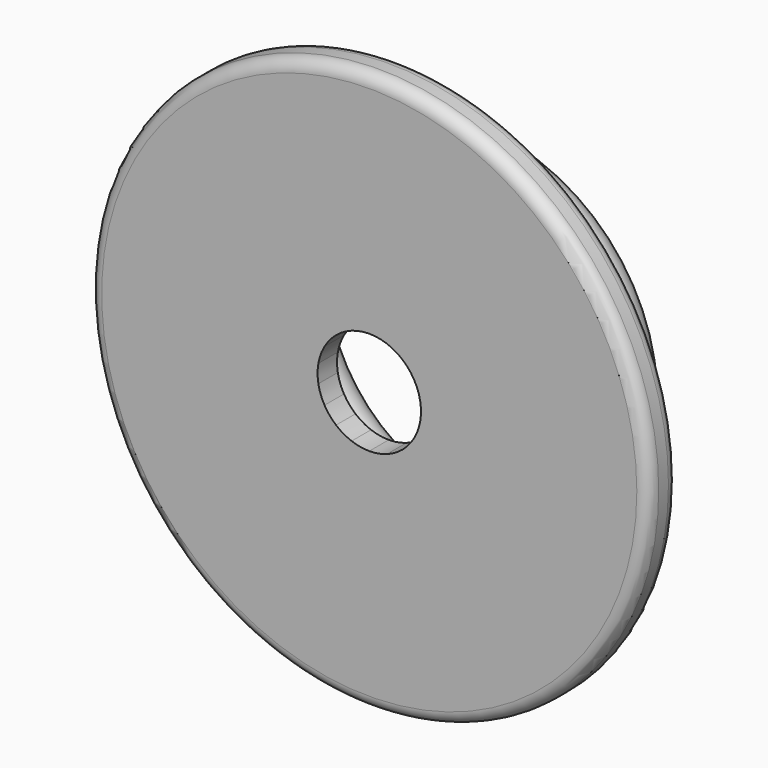
from build123d import *

# Parameters (mm, degrees)
F1_DEPTH = 10
F2_DEPTH = 2
F0_R     = 23
F3_DEPTH = 3
F4_DEPTH = 3.5
F5_R     = 1.6436802894
F7_R     = 1


with BuildPart() as f1:
    # F0 (on Front) → F1 (new body)
    with BuildSketch(Plane.XZ):
        with BuildLine():
            ThreePointArc((14.7721162952, -2.604722665), (14.9429204714, -1.3073361412), (15, 0))
            ThreePointArc((15, 0), (14.9429204714, 1.3073361412), (14.7721162952, 2.604722665))
            Line((14.7721162952, 2.604722665), (13.2949046657, 2.3442503985))
            ThreePointArc((13.2949046657, 2.3442503985), (13.4486284242, 1.1766025271), (13.5, 0))
            ThreePointArc((13.5, 0), (13.4486284242, -1.1766025271), (13.2949046657, -2.3442503985))
            Line((13.2949046657, -2.3442503985), (14.7721162952, -2.604722665))
        make_face()
    extrude(amount=-F1_DEPTH)



with BuildPart() as f1b:
    # F0 (on Front) → F1, piece 2 (new body)
    with BuildSketch(Plane.XZ):
        with BuildLine():
            Line((11.6913429511, 6.75), (12.9903810568, 7.5))
            ThreePointArc((12.9903810568, 7.5), (11.4906666468, 9.6418141453), (9.6418141453, 11.4906666468))
            Line((9.6418141453, 11.4906666468), (8.6776327308, 10.3415999821))
            ThreePointArc((8.6776327308, 10.3415999821), (10.3415999821, 8.6776327308), (11.6913429511, 6.75))
        make_face()
    extrude(amount=-F1_DEPTH)


with BuildPart() as f1c:
    # F0 (on Front) → F1, piece 3 (new body)
    with BuildSketch(Plane.XZ):
        with BuildLine():
            ThreePointArc((9.6418141453, -11.4906666468), (11.4906666468, -9.6418141453), (12.9903810568, -7.5))
            Line((12.9903810568, -7.5), (11.6913429511, -6.75))
            ThreePointArc((11.6913429511, -6.75), (10.3415999821, -8.6776327308), (8.6776327308, -10.3415999821))
            Line((8.6776327308, -10.3415999821), (9.6418141453, -11.4906666468))
        make_face()
    extrude(amount=-F1_DEPTH)


with BuildPart() as f1d:
    # F0 (on Front) → F1, piece 4 (new body)
    with BuildSketch(Plane.XZ):
        with BuildLine():
            Line((4.6172719349, 12.6858503806), (5.1303021499, 14.0953893118))
            ThreePointArc((5.1303021499, 14.0953893118), (3.8822856765, 14.4888873943), (2.604722665, 14.7721162952))
            ThreePointArc((2.604722665, 14.7721162952), (2.171185666, 14.842033311), (1.73578779, 14.8992295354))
            ThreePointArc((1.73578779, 14.8992295354), (0.869355212, 14.9747861926), (0, 15))
            Line((0, 15), (0, 13.5))
            ThreePointArc((0, 13.5), (2.3442503985, 13.2949046657), (4.6172719349, 12.6858503806))
        make_face()
    extrude(amount=-F1_DEPTH)


with BuildPart() as f1e:
    # F0 (on Front) → F1, piece 5 (new body)
    with BuildSketch(Plane.XZ):
        with BuildLine():
            ThreePointArc((0, -15), (2.604722665, -14.7721162952), (5.1303021499, -14.0953893118))
            Line((5.1303021499, -14.0953893118), (4.6172719349, -12.6858503806))
            ThreePointArc((4.6172719349, -12.6858503806), (2.3442503985, -13.2949046657), (0, -13.5))
            Line((0, -13.5), (0, -15))
        make_face()
    extrude(amount=-F1_DEPTH)


with BuildPart() as f1f:
    # F0 (on Front) → F1, piece 6 (new body)
    with BuildSketch(Plane.XZ):
        with BuildLine():
            ThreePointArc((-8.6776327308, 10.3415999821), (-6.75, 11.6913429511), (-4.6172719349, 12.6858503806))
            Line((-4.6172719349, 12.6858503806), (-5.1303021499, 14.0953893118))
            ThreePointArc((-5.1303021499, 14.0953893118), (-7.5, 12.9903810568), (-9.6418141453, 11.4906666468))
            Line((-9.6418141453, 11.4906666468), (-8.6776327308, 10.3415999821))
        make_face()
    extrude(amount=-F1_DEPTH)


with BuildPart() as f1g:
    # F0 (on Front) → F1, piece 7 (new body)
    with BuildSketch(Plane.XZ):
        with BuildLine():
            ThreePointArc((-13.2949046657, 2.3442503985), (-12.6858503806, 4.6172719349), (-11.6913429511, 6.75))
            Line((-11.6913429511, 6.75), (-12.9903810568, 7.5))
            ThreePointArc((-12.9903810568, 7.5), (-14.0953893118, 5.1303021499), (-14.7721162952, 2.604722665))
            Line((-14.7721162952, 2.604722665), (-13.2949046657, 2.3442503985))
        make_face()
    extrude(amount=-F1_DEPTH)


with BuildPart() as f1h:
    # F0 (on Front) → F1, piece 8 (new body)
    with BuildSketch(Plane.XZ):
        with BuildLine():
            ThreePointArc((-11.6913429511, -6.75), (-12.6858503806, -4.6172719349), (-13.2949046657, -2.3442503985))
            Line((-13.2949046657, -2.3442503985), (-14.7721162952, -2.604722665))
            ThreePointArc((-14.7721162952, -2.604722665), (-14.0953893118, -5.1303021499), (-12.9903810568, -7.5))
            Line((-12.9903810568, -7.5), (-11.6913429511, -6.75))
        make_face()
    extrude(amount=-F1_DEPTH)


with BuildPart() as f1i:
    # F0 (on Front) → F1, piece 9 (new body)
    with BuildSketch(Plane.XZ):
        with BuildLine():
            ThreePointArc((-4.6172719349, -12.6858503806), (-6.75, -11.6913429511), (-8.6776327308, -10.3415999821))
            Line((-8.6776327308, -10.3415999821), (-9.6418141453, -11.4906666468))
            ThreePointArc((-9.6418141453, -11.4906666468), (-7.5, -12.9903810568), (-5.1303021499, -14.0953893118))
            Line((-5.1303021499, -14.0953893118), (-4.6172719349, -12.6858503806))
        make_face()
    extrude(amount=-F1_DEPTH)


with BuildPart() as f1_1:
    add(f1.part)

    add(f1b.part)  # F2 merges F1b

    add(f1c.part)  # F2 merges F1c

    add(f1d.part)  # F2 merges F1d

    add(f1e.part)  # F2 merges F1e

    add(f1f.part)  # F2 merges F1f

    add(f1g.part)  # F2 merges F1g

    add(f1h.part)  # F2 merges F1h

    add(f1i.part)  # F2 merges F1i
    # F0 (on Front) → F2 (join)
    with BuildSketch(Plane.XZ):
        with BuildLine():
            ThreePointArc((-1.4535856091, 3.9936936383), (-0.7380047551, 4.1854329503), (0, 4.25))
            Line((0, 4.25), (0, 13.5))
            ThreePointArc((0, 13.5), (-2.3442503985, 13.2949046657), (-4.6172719349, 12.6858503806))
            Line((-4.6172719349, 12.6858503806), (-1.4535856091, 3.9936936383))
        make_face()
        with BuildLine():
            Line((1.4535856091, 3.9936936383), (4.6172719349, 12.6858503806))
            ThreePointArc((4.6172719349, 12.6858503806), (2.3442503985, 13.2949046657), (0, 13.5))
            Line((0, 13.5), (0, 4.25))
            ThreePointArc((0, 4.25), (0.7380047551, 4.1854329503), (1.4535856091, 3.9936936383))
        make_face()
        with BuildLine():
            Line((2.7318473412, 3.2556888833), (8.6776327308, 10.3415999821))
            ThreePointArc((8.6776327308, 10.3415999821), (6.75, 11.6913429511), (4.6172719349, 12.6858503806))
            Line((4.6172719349, 12.6858503806), (1.4535856091, 3.9936936383))
            ThreePointArc((1.4535856091, 3.9936936383), (2.125, 3.6806079661), (2.7318473412, 3.2556888833))
        make_face()
        with BuildLine():
            Line((3.6806079661, 2.125), (11.6913429511, 6.75))
            ThreePointArc((11.6913429511, 6.75), (10.3415999821, 8.6776327308), (8.6776327308, 10.3415999821))
            Line((8.6776327308, 10.3415999821), (2.7318473412, 3.2556888833))
            ThreePointArc((2.7318473412, 3.2556888833), (3.2556888833, 2.7318473412), (3.6806079661, 2.125))
        make_face()
        with BuildLine():
            Line((4.1854329503, 0.7380047551), (13.2949046657, 2.3442503985))
            ThreePointArc((13.2949046657, 2.3442503985), (12.6858503806, 4.6172719349), (11.6913429511, 6.75))
            Line((11.6913429511, 6.75), (3.6806079661, 2.125))
            ThreePointArc((3.6806079661, 2.125), (3.9936936383, 1.4535856091), (4.1854329503, 0.7380047551))
        make_face()
        with BuildLine():
            ThreePointArc((13.5, 0), (13.4486284242, 1.1766025271), (13.2949046657, 2.3442503985))
            Line((13.2949046657, 2.3442503985), (4.1854329503, 0.7380047551))
            ThreePointArc((4.1854329503, 0.7380047551), (4.2338274669, 0.3704119067), (4.25, 0))
            ThreePointArc((4.25, 0), (4.2338274669, -0.3704119067), (4.1854329503, -0.7380047551))
            Line((4.1854329503, -0.7380047551), (13.2949046657, -2.3442503985))
            ThreePointArc((13.2949046657, -2.3442503985), (13.4486284242, -1.1766025271), (13.5, 0))
        make_face()
        with BuildLine():
            ThreePointArc((11.6913429511, -6.75), (12.6858503806, -4.6172719349), (13.2949046657, -2.3442503985))
            Line((13.2949046657, -2.3442503985), (4.1854329503, -0.7380047551))
            ThreePointArc((4.1854329503, -0.7380047551), (3.9936936383, -1.4535856091), (3.6806079661, -2.125))
            Line((3.6806079661, -2.125), (11.6913429511, -6.75))
        make_face()
        with BuildLine():
            ThreePointArc((8.6776327308, -10.3415999821), (10.3415999821, -8.6776327308), (11.6913429511, -6.75))
            Line((11.6913429511, -6.75), (3.6806079661, -2.125))
            ThreePointArc((3.6806079661, -2.125), (3.2556888833, -2.7318473412), (2.7318473412, -3.2556888833))
            Line((2.7318473412, -3.2556888833), (8.6776327308, -10.3415999821))
        make_face()
        with BuildLine():
            ThreePointArc((4.6172719349, -12.6858503806), (6.75, -11.6913429511), (8.6776327308, -10.3415999821))
            Line((8.6776327308, -10.3415999821), (2.7318473412, -3.2556888833))
            ThreePointArc((2.7318473412, -3.2556888833), (2.125, -3.6806079661), (1.4535856091, -3.9936936383))
            Line((1.4535856091, -3.9936936383), (4.6172719349, -12.6858503806))
        make_face()
        with BuildLine():
            ThreePointArc((1.4535856091, -3.9936936383), (0.7380047551, -4.1854329503), (0, -4.25))
            Line((0, -4.25), (0, -13.5))
            ThreePointArc((0, -13.5), (2.3442503985, -13.2949046657), (4.6172719349, -12.6858503806))
            Line((4.6172719349, -12.6858503806), (1.4535856091, -3.9936936383))
        make_face()
        with BuildLine():
            ThreePointArc((0, -4.25), (-0.7380047551, -4.1854329503), (-1.4535856091, -3.9936936383))
            Line((-1.4535856091, -3.9936936383), (-4.6172719349, -12.6858503806))
            ThreePointArc((-4.6172719349, -12.6858503806), (-2.3442503985, -13.2949046657), (0, -13.5))
            Line((0, -13.5), (0, -4.25))
        make_face()
        with BuildLine():
            ThreePointArc((-1.4535856091, -3.9936936383), (-2.125, -3.6806079661), (-2.7318473412, -3.2556888833))
            Line((-2.7318473412, -3.2556888833), (-8.6776327308, -10.3415999821))
            ThreePointArc((-8.6776327308, -10.3415999821), (-6.75, -11.6913429511), (-4.6172719349, -12.6858503806))
            Line((-4.6172719349, -12.6858503806), (-1.4535856091, -3.9936936383))
        make_face()
        with BuildLine():
            ThreePointArc((-2.7318473412, -3.2556888833), (-3.2556888833, -2.7318473412), (-3.6806079661, -2.125))
            Line((-3.6806079661, -2.125), (-11.6913429511, -6.75))
            ThreePointArc((-11.6913429511, -6.75), (-10.3415999821, -8.6776327308), (-8.6776327308, -10.3415999821))
            Line((-8.6776327308, -10.3415999821), (-2.7318473412, -3.2556888833))
        make_face()
        with BuildLine():
            ThreePointArc((-3.6806079661, -2.125), (-3.9936936383, -1.4535856091), (-4.1854329503, -0.7380047551))
            Line((-4.1854329503, -0.7380047551), (-13.2949046657, -2.3442503985))
            ThreePointArc((-13.2949046657, -2.3442503985), (-12.6858503806, -4.6172719349), (-11.6913429511, -6.75))
            Line((-11.6913429511, -6.75), (-3.6806079661, -2.125))
        make_face()
        with BuildLine():
            ThreePointArc((-4.1854329503, -0.7380047551), (-4.25, 0), (-4.1854329503, 0.7380047551))
            Line((-4.1854329503, 0.7380047551), (-13.2949046657, 2.3442503985))
            ThreePointArc((-13.2949046657, 2.3442503985), (-13.5, 0), (-13.2949046657, -2.3442503985))
            Line((-13.2949046657, -2.3442503985), (-4.1854329503, -0.7380047551))
        make_face()
        with BuildLine():
            ThreePointArc((-4.1854329503, 0.7380047551), (-3.9936936383, 1.4535856091), (-3.6806079661, 2.125))
            Line((-3.6806079661, 2.125), (-11.6913429511, 6.75))
            ThreePointArc((-11.6913429511, 6.75), (-12.6858503806, 4.6172719349), (-13.2949046657, 2.3442503985))
            Line((-13.2949046657, 2.3442503985), (-4.1854329503, 0.7380047551))
        make_face()
        with BuildLine():
            ThreePointArc((-3.6806079661, 2.125), (-3.2556888833, 2.7318473412), (-2.7318473412, 3.2556888833))
            Line((-2.7318473412, 3.2556888833), (-8.6776327308, 10.3415999821))
            ThreePointArc((-8.6776327308, 10.3415999821), (-10.3415999821, 8.6776327308), (-11.6913429511, 6.75))
            Line((-11.6913429511, 6.75), (-3.6806079661, 2.125))
        make_face()
        with BuildLine():
            ThreePointArc((-2.7318473412, 3.2556888833), (-2.125, 3.6806079661), (-1.4535856091, 3.9936936383))
            Line((-1.4535856091, 3.9936936383), (-4.6172719349, 12.6858503806))
            ThreePointArc((-4.6172719349, 12.6858503806), (-6.75, 11.6913429511), (-8.6776327308, 10.3415999821))
            Line((-8.6776327308, 10.3415999821), (-2.7318473412, 3.2556888833))
        make_face()
    extrude(amount=-F2_DEPTH)

    # F0 (on Front) → F3 (join)
    with BuildSketch(Plane.XZ):
        Circle(F0_R)
        with BuildLine():
            ThreePointArc((14.7721162952, 2.604722665), (14.9429204714, 1.3073361412), (15, 0))
            ThreePointArc((15, 0), (14.9429204714, -1.3073361412), (14.7721162952, -2.604722665))
            ThreePointArc((14.7721162952, -2.604722665), (14.0953893118, -5.1303021499), (12.9903810568, -7.5))
            ThreePointArc((12.9903810568, -7.5), (11.4906666468, -9.6418141453), (9.6418141453, -11.4906666468))
            ThreePointArc((9.6418141453, -11.4906666468), (7.5, -12.9903810568), (5.1303021499, -14.0953893118))
            ThreePointArc((5.1303021499, -14.0953893118), (2.604722665, -14.7721162952), (0, -15))
            ThreePointArc((0, -15), (-2.604722665, -14.7721162952), (-5.1303021499, -14.0953893118))
            ThreePointArc((-5.1303021499, -14.0953893118), (-7.5, -12.9903810568), (-9.6418141453, -11.4906666468))
            ThreePointArc((-9.6418141453, -11.4906666468), (-11.4906666468, -9.6418141453), (-12.9903810568, -7.5))
            ThreePointArc((-12.9903810568, -7.5), (-14.0953893118, -5.1303021499), (-14.7721162952, -2.604722665))
            ThreePointArc((-14.7721162952, -2.604722665), (-15, 0), (-14.7721162952, 2.604722665))
            ThreePointArc((-14.7721162952, 2.604722665), (-14.0953893118, 5.1303021499), (-12.9903810568, 7.5))
            ThreePointArc((-12.9903810568, 7.5), (-11.4906666468, 9.6418141453), (-9.6418141453, 11.4906666468))
            ThreePointArc((-9.6418141453, 11.4906666468), (-7.5, 12.9903810568), (-5.1303021499, 14.0953893118))
            ThreePointArc((-5.1303021499, 14.0953893118), (-2.604722665, 14.7721162952), (0, 15))
            ThreePointArc((0, 15), (0.869355212, 14.9747861926), (1.73578779, 14.8992295354))
            ThreePointArc((1.73578779, 14.8992295354), (2.171185666, 14.842033311), (2.604722665, 14.7721162952))
            ThreePointArc((2.604722665, 14.7721162952), (3.8822856765, 14.4888873943), (5.1303021499, 14.0953893118))
            ThreePointArc((5.1303021499, 14.0953893118), (7.5, 12.9903810568), (9.6418141453, 11.4906666468))
            ThreePointArc((9.6418141453, 11.4906666468), (11.4906666468, 9.6418141453), (12.9903810568, 7.5))
            ThreePointArc((12.9903810568, 7.5), (14.0953893118, 5.1303021499), (14.7721162952, 2.604722665))
        make_face(mode=Mode.SUBTRACT)
    extrude(amount=-F3_DEPTH)

    # F0 (on Front) → F4 (join)
    with BuildSketch(Plane.XZ):
        with BuildLine():
            ThreePointArc((-13.2949046657, -2.3442503985), (-13.5, 0), (-13.2949046657, 2.3442503985))
            Line((-13.2949046657, 2.3442503985), (-14.7721162952, 2.604722665))
            ThreePointArc((-14.7721162952, 2.604722665), (-15, 0), (-14.7721162952, -2.604722665))
            Line((-14.7721162952, -2.604722665), (-13.2949046657, -2.3442503985))
        make_face()
        with BuildLine():
            ThreePointArc((-11.6913429511, 6.75), (-10.3415999821, 8.6776327308), (-8.6776327308, 10.3415999821))
            Line((-8.6776327308, 10.3415999821), (-9.6418141453, 11.4906666468))
            ThreePointArc((-9.6418141453, 11.4906666468), (-11.4906666468, 9.6418141453), (-12.9903810568, 7.5))
            Line((-12.9903810568, 7.5), (-11.6913429511, 6.75))
        make_face()
        with BuildLine():
            ThreePointArc((-4.6172719349, 12.6858503806), (-2.3442503985, 13.2949046657), (0, 13.5))
            Line((0, 13.5), (0, 15))
            ThreePointArc((0, 15), (-2.604722665, 14.7721162952), (-5.1303021499, 14.0953893118))
            Line((-5.1303021499, 14.0953893118), (-4.6172719349, 12.6858503806))
        make_face()
        with BuildLine():
            Line((8.6776327308, 10.3415999821), (9.6418141453, 11.4906666468))
            ThreePointArc((9.6418141453, 11.4906666468), (7.5, 12.9903810568), (5.1303021499, 14.0953893118))
            Line((5.1303021499, 14.0953893118), (4.6172719349, 12.6858503806))
            ThreePointArc((4.6172719349, 12.6858503806), (6.75, 11.6913429511), (8.6776327308, 10.3415999821))
        make_face()
        with BuildLine():
            Line((13.2949046657, 2.3442503985), (14.7721162952, 2.604722665))
            ThreePointArc((14.7721162952, 2.604722665), (14.0953893118, 5.1303021499), (12.9903810568, 7.5))
            Line((12.9903810568, 7.5), (11.6913429511, 6.75))
            ThreePointArc((11.6913429511, 6.75), (12.6858503806, 4.6172719349), (13.2949046657, 2.3442503985))
        make_face()
        with BuildLine():
            ThreePointArc((12.9903810568, -7.5), (14.0953893118, -5.1303021499), (14.7721162952, -2.604722665))
            Line((14.7721162952, -2.604722665), (13.2949046657, -2.3442503985))
            ThreePointArc((13.2949046657, -2.3442503985), (12.6858503806, -4.6172719349), (11.6913429511, -6.75))
            Line((11.6913429511, -6.75), (12.9903810568, -7.5))
        make_face()
        with BuildLine():
            ThreePointArc((5.1303021499, -14.0953893118), (7.5, -12.9903810568), (9.6418141453, -11.4906666468))
            Line((9.6418141453, -11.4906666468), (8.6776327308, -10.3415999821))
            ThreePointArc((8.6776327308, -10.3415999821), (6.75, -11.6913429511), (4.6172719349, -12.6858503806))
            Line((4.6172719349, -12.6858503806), (5.1303021499, -14.0953893118))
        make_face()
        with BuildLine():
            ThreePointArc((-5.1303021499, -14.0953893118), (-2.604722665, -14.7721162952), (0, -15))
            Line((0, -15), (0, -13.5))
            ThreePointArc((0, -13.5), (-2.3442503985, -13.2949046657), (-4.6172719349, -12.6858503806))
            Line((-4.6172719349, -12.6858503806), (-5.1303021499, -14.0953893118))
        make_face()
        with BuildLine():
            ThreePointArc((-8.6776327308, -10.3415999821), (-10.3415999821, -8.6776327308), (-11.6913429511, -6.75))
            Line((-11.6913429511, -6.75), (-12.9903810568, -7.5))
            ThreePointArc((-12.9903810568, -7.5), (-11.4906666468, -9.6418141453), (-9.6418141453, -11.4906666468))
            Line((-9.6418141453, -11.4906666468), (-8.6776327308, -10.3415999821))
        make_face()
    extrude(amount=-F4_DEPTH)

    # F7
    f7_edges = [f1_1.edges().sort_by_distance(p)[0] for p in [
        (-23, 3, 0),
        (-23, 0, 0),
    ]]
    fillet(f7_edges, radius=F7_R)


with BuildPart() as f6:
    # F5 (on Right) → F6 (revolve)
    with BuildSketch(Plane.YZ):
        with Locations((10.0005967543, -13.5725503787)):
            Circle(F5_R)
    revolve(axis=Axis((0, 18.1103013456, 0), (0, 1, 0)))


solid = Compound([f1_1.part, f6.part])
